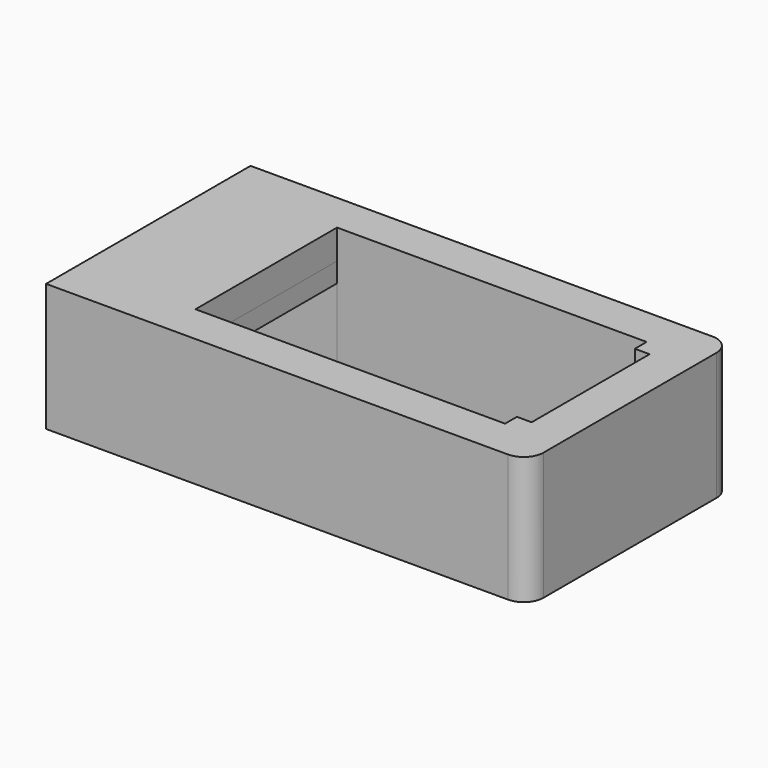
from build123d import *

# Parameters (mm, degrees)
F0_W          = 10
F0_H          = 2
F0_H_2        = 18
F1_DEPTH      = 2
F0_W_2        = 1.5
F0_H_3        = 1.5
F2_DEPTH      = 8
F3_W          = 15
F3_H          = 1.9559594506
F4_DEPTH      = 2
F3_W_2        = 1.5
F5_DEPTH      = 2
F5_DEPTH_BACK = 1.5
F6_DEPTH      = 8
F7_START      = -4.4440405494
F7_DEPTH      = 1.6
F8_R          = 2
F8_2_R        = 2
F10_DEPTH     = 10
F11_DEPTH     = 3


with BuildPart() as f1:
    # F0 (on Top) → F1 (new body)
    with BuildSketch(Plane.XY):
        with Locations((-16.5, 10)):
            Rectangle(F0_W, F0_H)
        with Locations((-16.5, -10)):
            Rectangle(F0_W, F0_H)
        with Locations((-16.5, 0)):
            Rectangle(F0_W, F0_H_2)
    extrude(amount=F1_DEPTH)

    # F0 (on Top) → F2 (join)
    with BuildSketch(Plane.XY):
        with Locations((-16.5, 10)):
            Rectangle(F0_W, F0_H)
        with Locations((-16.5, -10)):
            Rectangle(F0_W, F0_H)
    extrude(amount=-F2_DEPTH)

    # F3 (on face) → F4 (join)
    with BuildSketch(Plane(origin=(-21.5, 0, 0), x_dir=(0, -1, 0), z_dir=(-1, 0, 0))):
        with BuildLine():
            Line((-9, 0), (-9, -6.0440405494))
            Line((-9, -6.0440405494), (-7.5, -6.0440405494))
            Line((-7.5, -6.0440405494), (7.5, -6.0440405494))
            Line((7.5, -6.0440405494), (9, -6.0440405494))
            Line((9, -6.0440405494), (9, 0))
            Line((9, 0), (3.15, 0))
            ThreePointArc((3.15, 0), (3.7863961031, -0.2636038969), (4.05, -0.9))
            Line((4.05, -0.9), (4.05, -2.5242070224))
            ThreePointArc((4.05, -2.5242070224), (4.0468138033, -2.7821445636), (3.9705917564, -3.0285834538))
            Line((3.9705917564, -3.0285834538), (3.312223581, -4.0036350553))
            ThreePointArc((3.312223581, -4.0036350553), (2.9527146896, -4.3271018457), (2.4834570343, -4.4440405494))
            Line((2.4834570343, -4.4440405494), (-2.517703725, -4.4440405494))
            ThreePointArc((-2.517703725, -4.4440405494), (-2.9869613803, -4.3271018457), (-3.3464702717, -4.0036350553))
            Line((-3.3464702717, -4.0036350553), (-3.995889892, -3.0418363771))
            ThreePointArc((-3.995889892, -3.0418363771), (-4.1106105109, -2.8015443463), (-4.15, -2.5382013218))
            Line((-4.15, -2.5382013218), (-4.15, -1))
            ThreePointArc((-4.15, -1), (-3.8571067812, -0.2928932188), (-3.15, 0))
            Line((-3.15, 0), (-9, 0))
        make_face()
        Polygon((-9, -8), (-9, -6.0440405494), (-9, 0), (-3.15, 0), (3.15, 0), (9, 0), (9, -6.0440405494), (9, -8), (11, -8), (11, 2), (-11, 2), (-11, -8), align=None)
        with Locations((0, -7.0220202747)):
            Rectangle(F3_W, F3_H)
    extrude(amount=F4_DEPTH)

    # F3 (on face) → F5 (join, two sides)
    with BuildSketch(Plane(origin=(-21.5, 0, 0), x_dir=(0, -1, 0), z_dir=(-1, 0, 0))) as f5_sk:
        with Locations((8.25, -7.0220202747)):
            Rectangle(F3_W_2, F3_H)
        with Locations((-8.25, -7.0220202747)):
            Rectangle(F3_W_2, F3_H)
    extrude(amount=F5_DEPTH)
    extrude(f5_sk.sketch, amount=-F5_DEPTH_BACK)

    # F8
    f8_edges = [f1.edges().sort_by_distance(p)[0] for p in [
        (-23.5, 11, -3),
        (-23.5, -11, -3),
        (-11.5, 11, -3),
        (-11.5, -11, -3),
    ]]
    fillet(f8_edges, radius=F8_R)


with BuildPart() as f1b:
    # F0 (on Top) → F1, piece 2 (new body)
    with BuildSketch(Plane.XY):
        with Locations((20.75, -10)):
            Rectangle(F0_W_2, F0_H)
        with Locations((20.75, 8.25)):
            Rectangle(F0_W_2, F0_H_3)
        with Locations((20.75, -8.25)):
            Rectangle(F0_W_2, F0_H_3)
        Polygon((21.5, -7.5), (21.5, -9), (21.5, -11), (23.5, -11), (23.5, 11), (21.5, 11), (21.5, 9), (21.5, 7.5), align=None)
        with Locations((20.75, 10)):
            Rectangle(F0_W_2, F0_H)
    extrude(amount=F1_DEPTH)

    # F0 (on Top) → F6 (join, through all)
    with BuildSketch(Plane.XY):
        Polygon((21.5, -7.5), (21.5, -9), (21.5, -11), (23.5, -11), (23.5, 11), (21.5, 11), (21.5, 9), (21.5, 7.5), align=None)
        with Locations((20.75, -10)):
            Rectangle(F0_W_2, F0_H)
        with Locations((20.75, 10)):
            Rectangle(F0_W_2, F0_H)
        with Locations((20.75, -8.25)):
            Rectangle(F0_W_2, F0_H_3)
        with Locations((20.75, 8.25)):
            Rectangle(F0_W_2, F0_H_3)
    extrude(amount=-F6_DEPTH)

    # F0 (on Top) → F7 (cut)
    with BuildSketch(Plane.XY.offset(F7_START)):
        with Locations((20.75, -8.25)):
            Rectangle(F0_W_2, F0_H_3)
        with Locations((20.75, 8.25)):
            Rectangle(F0_W_2, F0_H_3)
    extrude(amount=-F7_DEPTH, mode=Mode.SUBTRACT)

    # F8#2
    f8_2_edges = [f1b.edges().sort_by_distance(p)[0] for p in [
        (23.5, 11, -3),
        (23.5, -11, -3),
    ]]
    fillet(f8_2_edges, radius=F8_2_R)


with BuildPart() as f10:
    # F9 (on face) → F10 (new body, through all)
    with BuildSketch(Plane.XY.offset(2)):
        with BuildLine():
            ThreePointArc((-21.5, -11), (-22.9142135624, -10.4142135624), (-23.5, -9))
            Line((-23.5, -9), (-23.5, -13))
            Line((-23.5, -13), (23.5, -13))
            ThreePointArc((23.5, -13), (24.9142135624, -12.4142135624), (25.5, -11))
            Line((25.5, -11), (25.5, 0))
            Line((25.5, 0), (25.5, 11))
            ThreePointArc((25.5, 11), (24.9142135624, 12.4142135624), (23.5, 13))
            Line((23.5, 13), (-23.5, 13))
            Line((-23.5, 13), (-23.5, 9))
            ThreePointArc((-23.5, 9), (-22.9142135624, 10.4142135624), (-21.5, 11))
            Line((-21.5, 11), (-13.5, 11))
            Line((-13.5, 11), (20, 11))
            Line((20, 11), (21.5, 11))
            ThreePointArc((21.5, 11), (22.9142135624, 10.4142135624), (23.5, 9))
            Line((23.5, 9), (23.5, 0))
            Line((23.5, 0), (23.5, -9))
            ThreePointArc((23.5, -9), (22.9142135624, -10.4142135624), (21.5, -11))
            Line((21.5, -11), (20, -11))
            Line((20, -11), (-13.5, -11))
            Line((-13.5, -11), (-21.5, -11))
        make_face()
        with BuildLine():
            ThreePointArc((-11.5, -9), (-12.0857864376, -10.4142135624), (-13.5, -11))
            Line((-13.5, -11), (20, -11))
            Line((20, -11), (20, -9))
            Line((20, -9), (-11.5, -9))
        make_face()
        with BuildLine():
            Line((20, 11), (-13.5, 11))
            ThreePointArc((-13.5, 11), (-12.0857864376, 10.4142135624), (-11.5, 9))
            Line((-11.5, 9), (20, 9))
            Line((20, 9), (20, 11))
        make_face()
    extrude(amount=-F10_DEPTH)

    # F9 (on face) → F11 (join)
    with BuildSketch(Plane.XY.offset(2)):
        with BuildLine():
            ThreePointArc((-21.5, -11), (-22.9142135624, -10.4142135624), (-23.5, -9))
            Line((-23.5, -9), (-23.5, -13))
            Line((-23.5, -13), (23.5, -13))
            ThreePointArc((23.5, -13), (24.9142135624, -12.4142135624), (25.5, -11))
            Line((25.5, -11), (25.5, 0))
            Line((25.5, 0), (25.5, 11))
            ThreePointArc((25.5, 11), (24.9142135624, 12.4142135624), (23.5, 13))
            Line((23.5, 13), (-23.5, 13))
            Line((-23.5, 13), (-23.5, 9))
            ThreePointArc((-23.5, 9), (-22.9142135624, 10.4142135624), (-21.5, 11))
            Line((-21.5, 11), (-13.5, 11))
            Line((-13.5, 11), (20, 11))
            Line((20, 11), (21.5, 11))
            ThreePointArc((21.5, 11), (22.9142135624, 10.4142135624), (23.5, 9))
            Line((23.5, 9), (23.5, 0))
            Line((23.5, 0), (23.5, -9))
            ThreePointArc((23.5, -9), (22.9142135624, -10.4142135624), (21.5, -11))
            Line((21.5, -11), (20, -11))
            Line((20, -11), (-13.5, -11))
            Line((-13.5, -11), (-21.5, -11))
        make_face()
        with BuildLine():
            Line((20, -9), (20, -11))
            Line((20, -11), (21.5, -11))
            ThreePointArc((21.5, -11), (22.9142135624, -10.4142135624), (23.5, -9))
            Line((23.5, -9), (23.5, 0))
            Line((23.5, 0), (23.5, 9))
            ThreePointArc((23.5, 9), (22.9142135624, 10.4142135624), (21.5, 11))
            Line((21.5, 11), (20, 11))
            Line((20, 11), (20, 9))
            Line((20, 9), (20, 7.5))
            Line((20, 7.5), (21.5, 7.5))
            Line((21.5, 7.5), (21.5, -7.5))
            Line((21.5, -7.5), (20, -7.5))
            Line((20, -7.5), (20, -9))
        make_face()
        with BuildLine():
            Line((-23.5, 9), (-23.5, -9))
            ThreePointArc((-23.5, -9), (-22.9142135624, -10.4142135624), (-21.5, -11))
            Line((-21.5, -11), (-13.5, -11))
            ThreePointArc((-13.5, -11), (-12.0857864376, -10.4142135624), (-11.5, -9))
            Line((-11.5, -9), (-11.5, 9))
            ThreePointArc((-11.5, 9), (-12.0857864376, 10.4142135624), (-13.5, 11))
            Line((-13.5, 11), (-21.5, 11))
            ThreePointArc((-21.5, 11), (-22.9142135624, 10.4142135624), (-23.5, 9))
        make_face()
        with BuildLine():
            Line((20, 11), (-13.5, 11))
            ThreePointArc((-13.5, 11), (-12.0857864376, 10.4142135624), (-11.5, 9))
            Line((-11.5, 9), (20, 9))
            Line((20, 9), (20, 11))
        make_face()
        with BuildLine():
            ThreePointArc((-11.5, -9), (-12.0857864376, -10.4142135624), (-13.5, -11))
            Line((-13.5, -11), (20, -11))
            Line((20, -11), (20, -9))
            Line((20, -9), (-11.5, -9))
        make_face()
    extrude(amount=F11_DEPTH)


solid = Compound([f1.part, f1b.part, f10.part])
